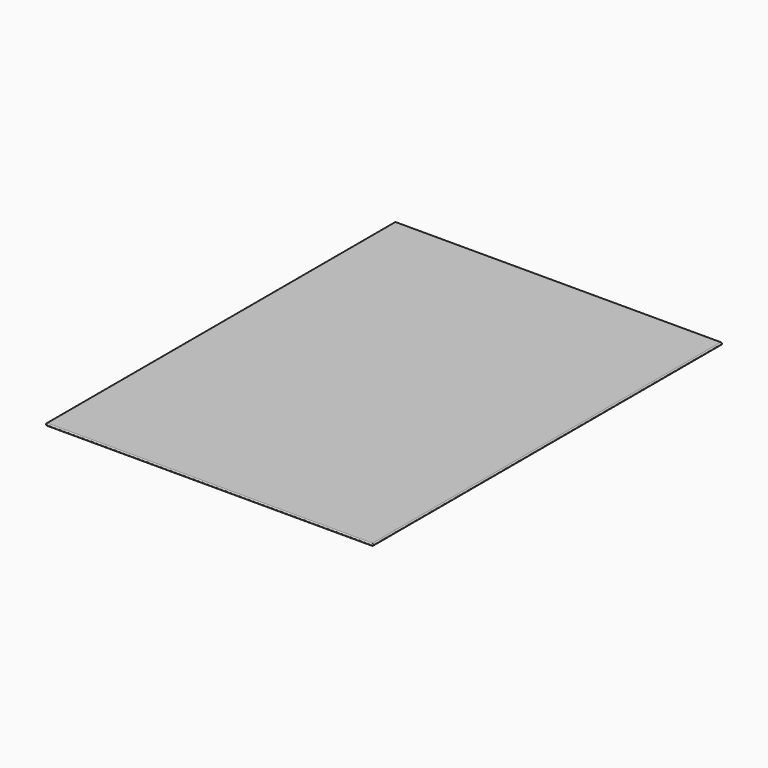
from build123d import *

# Parameters (mm, degrees)
F0_W     = 147.701
F0_H     = 197.358
F1_DEPTH = 1.016
F2_R     = 0.50799


# Not quite as in the source:
# - a fillet or chamfer is up to 0.001 mm smaller than in the source, because OpenCascade refuses the exact size


with BuildPart() as f1:
    # F0 (on Top) → F1 (new body)
    with BuildSketch(Plane.XY):
        Rectangle(F0_W, F0_H)
    extrude(amount=F1_DEPTH)

    # F2 (radius 0.508 in the source; OpenCascade refuses exactly that, so slightly less here)
    f2_edges = [f1.edges().sort_by_distance(p)[0] for p in [
        (73.8505, -98.679, 0.508),
        (73.8505, 98.679, 0.508),
        (73.8505, 0, 0),
        (73.8505, 0, 1.016),
        (-73.8505, 98.679, 0.508),
        (0, 98.679, 0),
        (0, 98.679, 1.016),
        (-73.8505, -98.679, 0.508),
        (-73.8505, 0, 0),
        (-73.8505, 0, 1.016),
        (0, -98.679, 0),
        (0, -98.679, 1.016),
    ]]
    fillet(f2_edges, radius=F2_R)


solid = f1.part
